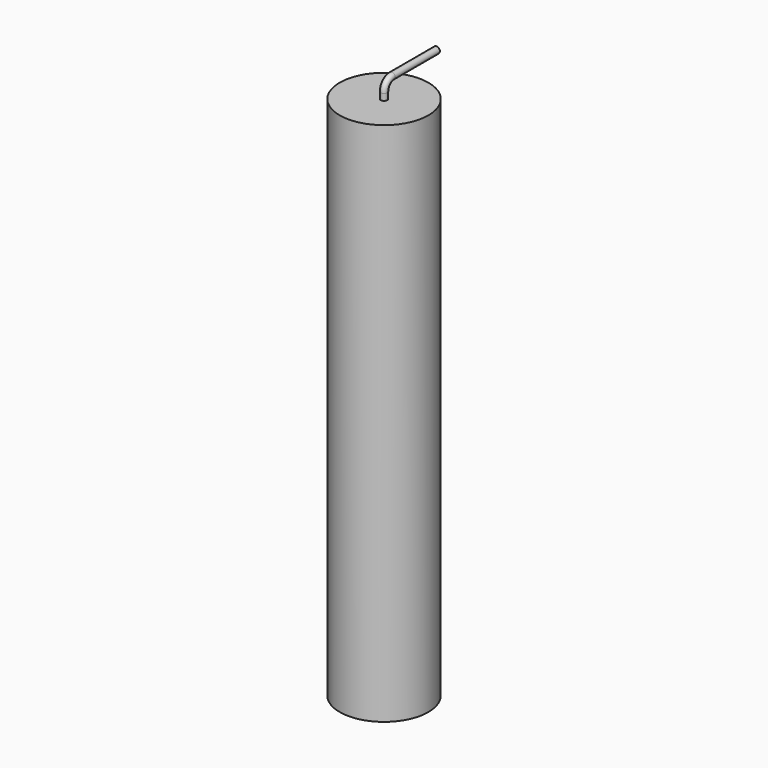
from build123d import *

# Parameters (mm, degrees)
F0_R      = 135
F1_DEPTH  = 1600
F2_R      = 10
F6_DEPTH  = 5
F5_R      = 10
F7_DEPTH  = 25
F8_T      = -3
F9_R      = 8.5
F10_DEPTH = 50
F11_R     = 10
F11_R_2   = 7.5


with BuildPart() as f1:
    # F0 (on Top) → F1 (new body)
    with BuildSketch(Plane.XY):
        Circle(F0_R)
    extrude(amount=F1_DEPTH)

    # F2 (on face) → F6 (join)
    with BuildSketch(Plane.XY.offset(1600)):
        Circle(F2_R)
    extrude(amount=F6_DEPTH)

    # F5 (on offset) → F7 (join)
    with BuildSketch(Plane.XZ.offset(-125)):
        with Locations((0, 1565)):
            Circle(F5_R)
    extrude(amount=-F7_DEPTH)

    # F8
    f8_openings = [f1.faces().sort_by_distance(p)[0] for p in [
        (0, 0, 0),
    ]]
    offset(amount=F8_T, openings=f8_openings, kind=Kind.INTERSECTION)

    # F9 (on face) → F10 (cut)
    with BuildSketch(Plane(origin=(0, 150, 0), x_dir=(-1, 0, 0), z_dir=(0, 1, 0))):
        with Locations((0, 1565)):
            Circle(F9_R)
    extrude(amount=-F10_DEPTH, mode=Mode.SUBTRACT)

    # F12: sweep along a path in F3
    with BuildLine(Plane.YZ) as f12_path:
        Line((0, 1600), (0, 1620))
        ThreePointArc((0, 1620), (8.7867965644, 1641.2132034356), (30, 1650))
        Line((30, 1650), (200, 1650))
    # F11 (on face) → F12 (sweep)
    with BuildSketch(Plane.XY.offset(1605)):
        Circle(F11_R)
        Circle(F11_R_2, mode=Mode.SUBTRACT)
    sweep(path=f12_path.line)


solid = f1.part
